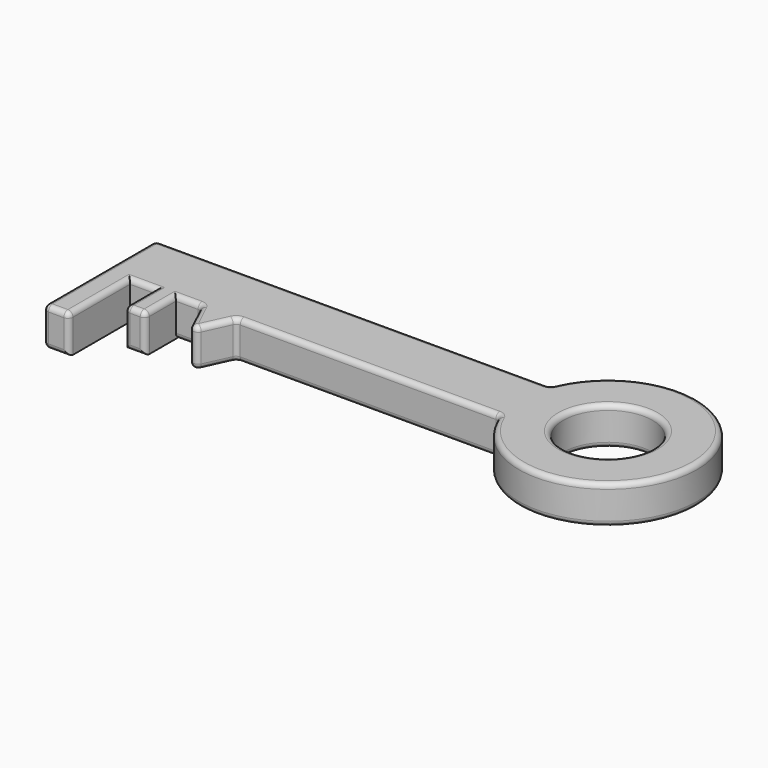
from build123d import *

# Parameters (mm, degrees)
F0_R     = 17.5
F0_W     = 8
F0_H     = 15
F0_W_2   = 10
F0_H_2   = 30
F1_DEPTH = 15
F2_R     = 2


with BuildPart() as f1:
    # F0 (on Top) → F1 (new body)
    with BuildSketch(Plane.XY):
        with BuildLine():
            Line((67.8651795072, 58.3995857492), (-87.1348204928, 58.3995857492))
            Line((-87.1348204928, 58.3995857492), (-87.1348204928, 33.3995857492))
            Line((-87.1348204928, 33.3995857492), (-77.1348204928, 33.3995857492))
            Line((-77.1348204928, 33.3995857492), (-67.1348204928, 33.3995857492))
            Line((-67.1348204928, 33.3995857492), (-59.1348204928, 33.3995857492))
            Line((-59.1348204928, 33.3995857492), (-49.1348204928, 33.3995857492))
            Line((-49.1348204928, 33.3995857492), (-35.1348204928, 33.3995857492))
            Line((-35.1348204928, 33.3995857492), (67.8651795072, 33.3995857492))
            ThreePointArc((67.8651795072, 33.3995857492), (135.5569215837, 45.8995857492), (67.8651795072, 58.3995857492))
        make_face()
        with Locations((100.5569215837, 45.8995857492)):
            Circle(F0_R, mode=Mode.SUBTRACT)
        with Locations((-63.1348204928, 25.8995857492)):
            Rectangle(F0_W, F0_H)
        Polygon((-42.0509860516, 18.3606874198), (-35.1348204928, 33.3995857492), (-49.1348204928, 33.3995857492), align=None)
        with Locations((-82.1348204928, 18.3995857492)):
            Rectangle(F0_W_2, F0_H_2)
    extrude(amount=F1_DEPTH)

    # F2
    f2_edges = [f1.edges().sort_by_distance(p)[0] for p in [
        (-54.13482, 33.399586, 15),
        (-9.63482, 58.399586, 15),
        (-87.13482, 30.899586, 15),
        (-82.13482, 3.399586, 15),
        (-77.13482, 18.399586, 15),
        (-72.13482, 33.399586, 15),
        (-67.13482, 25.899586, 15),
        (-63.13482, 18.399586, 15),
        (-59.13482, 25.899586, 15),
        (-45.592903, 25.880137, 15),
        (-38.592903, 25.880137, 15),
        (16.36518, 33.399586, 15),
        (135.556922, 45.899586, 15),
        (83.056922, 45.899586, 15),
        (135.556922, 45.899586, 0),
        (67.86518, 33.399586, 7.5),
        (67.86518, 58.399586, 7.5),
        (-87.13482, 58.399586, 7.5),
        (-9.63482, 58.399586, 0),
        (-87.13482, 3.399586, 7.5),
        (-87.13482, 30.899586, 0),
        (-77.13482, 3.399586, 7.5),
        (-59.13482, 18.399586, 7.5),
        (-49.13482, 33.399586, 7.5),
        (-42.050986, 18.360687, 7.5),
        (-45.592903, 25.880137, 0),
        (-35.13482, 33.399586, 7.5),
        (-82.13482, 3.399586, 0),
        (-67.13482, 18.399586, 7.5),
        (83.056922, 45.899586, 0),
        (-63.13482, 18.399586, 0),
        (-38.592903, 25.880137, 0),
        (16.36518, 33.399586, 0),
        (-54.13482, 33.399586, 0),
    ]]
    fillet(f2_edges, radius=F2_R)


solid = f1.part
